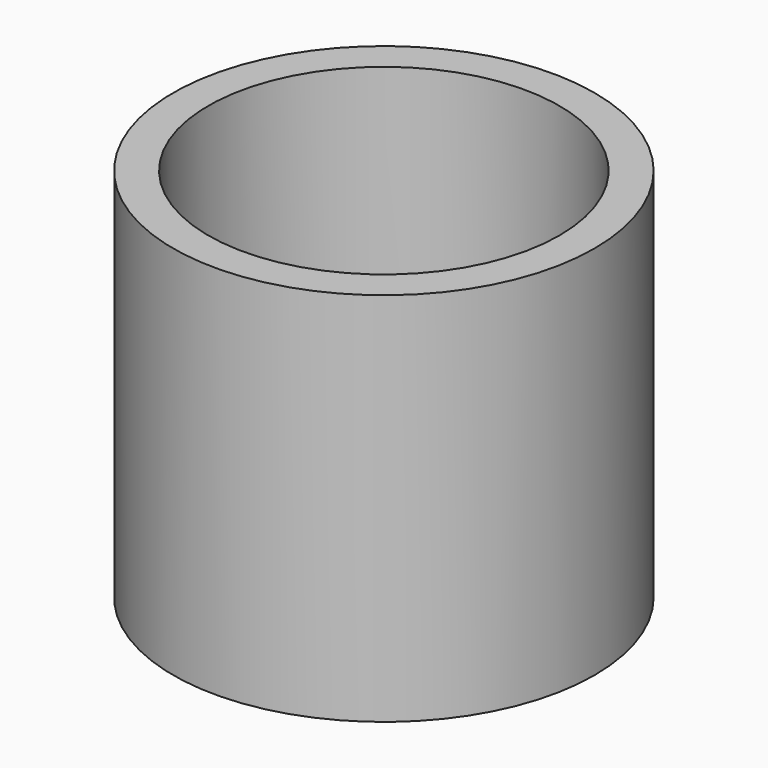
from build123d import *

# Parameters (mm, degrees)
F2_R     = 25.4
F2_R_2   = 17.78
F3_DEPTH = 33.02
F4_DEPTH = 60.96
F5_W     = 2.54
F5_H     = 16.6851995905
F5_H_2   = 2.54
F5_W_2   = 16.7025072155
F6_DEPTH = 25.4254
F8_DEPTH = 25.4254


# Not quite as in the source:
# - a feature names something its author has since deleted; it is built from what else it names


with BuildPart() as f1:
    # F0 (on Front) → F1 (revolve)
    with BuildSketch(Plane.XZ):
        with BuildLine():
            Line((30.48, 60.96), (0, 60.96))
            Line((0, 60.96), (0, 0))
            ThreePointArc((0, 0), (15.5534533119, 1.861565962), (30.48, 6.6127281069))
            Line((30.48, 6.6127281069), (30.48, 60.96))
        make_face()
    revolve(axis=Axis((0, 0, 30.48), (0, 0, -1)))

    # F2 (on face) → F3 (cut)
    with BuildSketch(Plane.XY.offset(60.96)):
        Circle(F2_R)
        Circle(F2_R_2, mode=Mode.SUBTRACT)
    extrude(amount=-F3_DEPTH, mode=Mode.SUBTRACT)

    # F4 (cut): a face of the model
    f4_faces = [f1.faces().sort_by_distance(p)[0] for p in [
        (0, 0, 60.96),
    ]]
    extrude(f4_faces, amount=-F4_DEPTH, mode=Mode.SUBTRACT)


with BuildPart() as f6:
    # F5 (on face) → F6 (new body)
    with BuildSketch(Plane.XY.offset(27.94)):
        with Locations((0, -9.6125997952)):
            Rectangle(F5_W, F5_H)
        Rectangle(F5_W, F5_H_2)
        with Locations((9.6212536077, 0)):
            Rectangle(F5_W_2, F5_H_2)
        with Locations((-9.6212536077, 0)):
            Rectangle(F5_W_2, F5_H_2)
        with Locations((0, 9.6125997952)):
            Rectangle(F5_W, F5_H)
    extrude(amount=-F6_DEPTH)

    # F7 (on face) → F8 (join)
    with BuildSketch(Plane.XY.offset(27.94)):
        with BuildLine():
            ThreePointArc((0, -10.2025506097), (7.2142927215, -7.2142927215), (10.2025506097, 0))
            ThreePointArc((10.2025506097, 0), (-7.2142927215, 7.2142927215), (0, -10.2025506097))
        make_face()
    extrude(amount=-F8_DEPTH)


solid = Compound([f1.part, f6.part])
